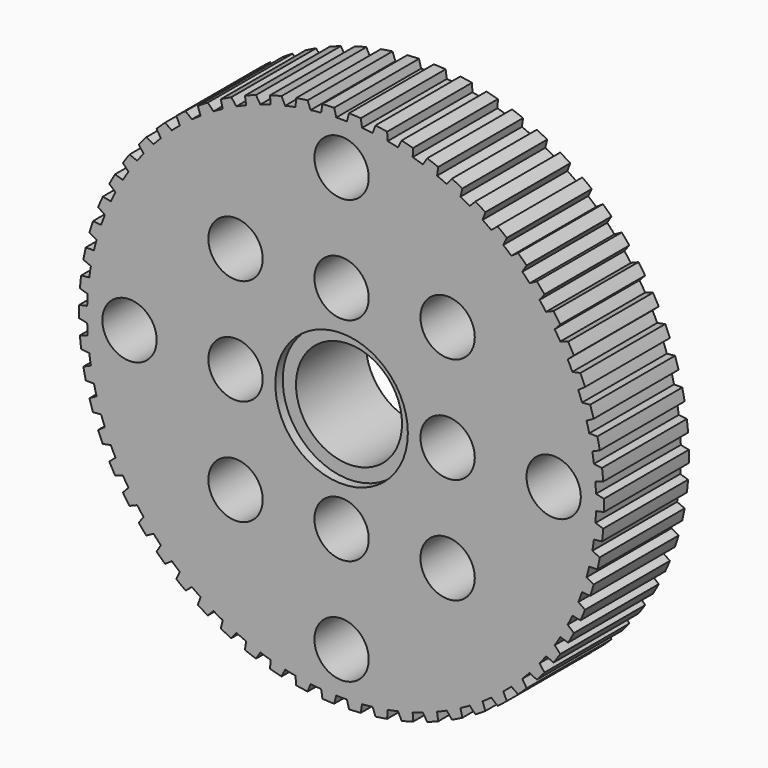
from build123d import *

# Parameters (mm, degrees)
F0_R            = 19.8
F0_R_2          = 2.05
F0_R_3          = 4
F1_DEPTH        = 4
F2_R            = 5
F3_DEPTH        = 0.7
F5_DEPTH        = 25.4
F5_COPIES_COUNT = 62


# Not quite as in the source:
# - a pattern or mirror of a feature is missing from the dataset's text; its kind, count and spacing are read off the source's solid


with BuildPart() as f1:
    # F0 (on Front) → F1 (new body, symmetric)
    with BuildSketch(Plane.XZ):
        Circle(F0_R)
        with Locations((-8, -8)):
            Circle(F0_R_2, mode=Mode.SUBTRACT)
        with Locations((0, -16)):
            Circle(F0_R_2, mode=Mode.SUBTRACT)
        with Locations((0, -8)):
            Circle(F0_R_2, mode=Mode.SUBTRACT)
        with Locations((8, -8)):
            Circle(F0_R_2, mode=Mode.SUBTRACT)
        with Locations((-16, 0)):
            Circle(F0_R_2, mode=Mode.SUBTRACT)
        with Locations((-8, 0)):
            Circle(F0_R_2, mode=Mode.SUBTRACT)
        with Locations((-8, 8)):
            Circle(F0_R_2, mode=Mode.SUBTRACT)
        Circle(F0_R_3, mode=Mode.SUBTRACT)
        with Locations((8, 0)):
            Circle(F0_R_2, mode=Mode.SUBTRACT)
        with Locations((0, 8)):
            Circle(F0_R_2, mode=Mode.SUBTRACT)
        with Locations((8, 8)):
            Circle(F0_R_2, mode=Mode.SUBTRACT)
        with Locations((16, 0)):
            Circle(F0_R_2, mode=Mode.SUBTRACT)
        with Locations((0, 16)):
            Circle(F0_R_2, mode=Mode.SUBTRACT)
    extrude(amount=F1_DEPTH, both=True)

    # F2 (on face) → F3 (cut)
    with BuildSketch(Plane.XZ.offset(4)):
        Circle(F2_R)
    f3 = extrude(amount=-F3_DEPTH, mode=Mode.SUBTRACT)

    # F3_copies: F3 across plane
    add(f3.mirror(Plane.ZX), mode=Mode.SUBTRACT)

    # F4 (on face) → F5 (cut)
    with BuildSketch(Plane.XZ.offset(4)):
        with BuildLine():
            Line((1.0817075249, 21.74), (-1.0817075249, 21.74))
            Line((-1.0817075249, 21.74), (-0.4, 19.1958328811))
            ThreePointArc((-0.4, 19.1958328811), (0, 19.2), (0.4, 19.1958328811))
            Line((0.4, 19.1958328811), (1.0817075249, 21.74))
        make_face()
    f5 = extrude(amount=-F5_DEPTH, mode=Mode.SUBTRACT)

    # F5_copies: F5 ×62 about axis
    f5_copies_axis = Axis((0, 0, 0), (0, 1, 0))
    for i in range(1, F5_COPIES_COUNT):
        add(f5.rotate(f5_copies_axis, i * 360 / F5_COPIES_COUNT), mode=Mode.SUBTRACT)


solid = f1.part
